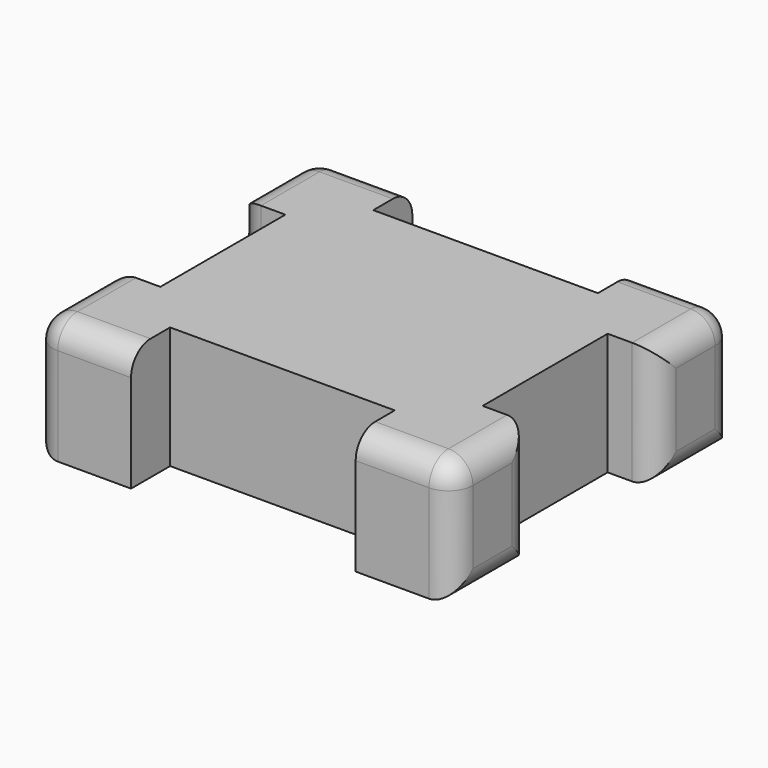
from build123d import *

# Parameters (mm, degrees)
F0_W         = 10
F0_H         = 10
F1_DEPTH     = 25
F2_T         = -2.5
F3_T1_DEPTH  = 27.5
F3_T3_DEPTH  = 27.5
F3_T5_DEPTH  = 27.5
F3_T7_DEPTH  = 27.5
F3_T9_DEPTH  = 32.5
F3_T11_DEPTH = 50
F3_T13_DEPTH = 45
F3_T15_DEPTH = 45
F3_S19_W     = 5
F3_S19_H     = 5
F3_T20_DEPTH = 5
F3_S25_W     = 5
F3_S25_H     = 5
F3_T26_DEPTH = 5
F3_S31_W     = 5
F3_S31_H     = 5
F3_T32_DEPTH = 5
F3_S37_W     = 5
F3_S37_H     = 5
F3_T38_DEPTH = 5


# Not quite as in the source:
# - a fillet or chamfer that OpenCascade refuses, or shapes differently, is made with other operations: its cross-section is extruded or revolved along the edge and cut away or added


with BuildPart() as f1:
    # F0 (on Top) → F1 (new body)
    with BuildSketch(Plane.XY):
        Polygon((-33, 16), (-33, 26), (-23, 26), (-23, 36), (-43, 36), (-43, 16), align=None)
        with Locations((-28, 21)):
            Rectangle(F0_W, F0_H)
        Polygon((23, 26), (-23, 26), (-23, 16), (-33, 16), (-33, -16), (-23, -16), (-23, -26), (23, -26), (23, -16), (33, -16), (33, 16), (23, 16), align=None)
        Polygon((23, 36), (23, 26), (33, 26), (33, 16), (43, 16), (43, 36), align=None)
        with Locations((28, 21)):
            Rectangle(F0_W, F0_H)
        with Locations((-28, -21)):
            Rectangle(F0_W, F0_H)
        Polygon((-33, -26), (-33, -16), (-43, -16), (-43, -36), (-23, -36), (-23, -26), align=None)
        Polygon((43, -16), (33, -16), (33, -26), (23, -26), (23, -36), (43, -36), align=None)
        with Locations((28, -21)):
            Rectangle(F0_W, F0_H)
    extrude(amount=F1_DEPTH)

    # F2
    f2_openings = [f1.faces().sort_by_distance(p)[0] for p in [
        (0, 0, 0),
    ]]
    offset(amount=F2_T, openings=f2_openings, kind=Kind.INTERSECTION)

    # F3: fillet of radius 5 on 20 edges, made by hand

    # F3_s2 → F3_t1 (cut)
    with BuildSketch(Plane.YZ.offset(-38)):
        with BuildLine():
            ThreePointArc((36, 20), (34.5355339059, 23.5355339059), (31, 25))
            Line((31, 25), (36, 25))
            Line((36, 25), (36, 20))
        make_face()
        with BuildLine():
            ThreePointArc((-36, 20), (-34.5355339059, 23.5355339059), (-31, 25))
            Line((-31, 25), (-36, 25))
            Line((-36, 25), (-36, 20))
        make_face()
    extrude(amount=F3_T1_DEPTH, mode=Mode.SUBTRACT)

    # F3_s4 → F3_t3 (cut)
    with BuildSketch(Plane.YZ.offset(10.5)):
        with BuildLine():
            ThreePointArc((-36, 20), (-34.5355339059, 23.5355339059), (-31, 25))
            Line((-31, 25), (-36, 25))
            Line((-36, 25), (-36, 20))
        make_face()
        with BuildLine():
            ThreePointArc((36, 20), (34.5355339059, 23.5355339059), (31, 25))
            Line((31, 25), (36, 25))
            Line((36, 25), (36, 20))
        make_face()
    extrude(amount=F3_T3_DEPTH, mode=Mode.SUBTRACT)

    # F3_s6 → F3_t5 (cut)
    with BuildSketch(Plane.XZ.offset(-31)):
        with BuildLine():
            ThreePointArc((43, 20), (41.5355339059, 23.5355339059), (38, 25))
            Line((38, 25), (43, 25))
            Line((43, 25), (43, 20))
        make_face()
        with BuildLine():
            ThreePointArc((-43, 20), (-41.5355339059, 23.5355339059), (-38, 25))
            Line((-38, 25), (-43, 25))
            Line((-43, 25), (-43, 20))
        make_face()
    extrude(amount=F3_T5_DEPTH, mode=Mode.SUBTRACT)

    # F3_s8 → F3_t7 (cut)
    with BuildSketch(Plane.XZ.offset(3.5)):
        with BuildLine():
            ThreePointArc((43, 20), (41.5355339059, 23.5355339059), (38, 25))
            Line((38, 25), (43, 25))
            Line((43, 25), (43, 20))
        make_face()
        with BuildLine():
            ThreePointArc((-43, 20), (-41.5355339059, 23.5355339059), (-38, 25))
            Line((-38, 25), (-43, 25))
            Line((-43, 25), (-43, 20))
        make_face()
    extrude(amount=F3_T7_DEPTH, mode=Mode.SUBTRACT)

    # F3_s10 → F3_t9 (cut)
    with BuildSketch(Plane.XY.offset(-12.5)):
        with BuildLine():
            ThreePointArc((-38, 36), (-41.5355339059, 34.5355339059), (-43, 31))
            Line((-43, 31), (-43, 36))
            Line((-43, 36), (-38, 36))
        make_face()
        with BuildLine():
            ThreePointArc((43, 31), (41.5355339059, 34.5355339059), (38, 36))
            Line((38, 36), (43, 36))
            Line((43, 36), (43, 31))
        make_face()
        with BuildLine():
            ThreePointArc((38, -36), (41.5355339059, -34.5355339059), (43, -31))
            Line((43, -31), (43, -36))
            Line((43, -36), (38, -36))
        make_face()
        with BuildLine():
            ThreePointArc((-43, -31), (-41.5355339059, -34.5355339059), (-38, -36))
            Line((-38, -36), (-43, -36))
            Line((-43, -36), (-43, -31))
        make_face()
    extrude(amount=F3_T9_DEPTH, mode=Mode.SUBTRACT)

    # F3_s12 → F3_t11 (cut)
    with BuildSketch(Plane.XY.offset(-12.5)):
        with BuildLine():
            ThreePointArc((-43, 21), (-41.5355339059, 17.4644660941), (-38, 16))
            Line((-38, 16), (-43, 16))
            Line((-43, 16), (-43, 21))
        make_face()
        with BuildLine():
            ThreePointArc((38, 16), (41.5355339059, 17.4644660941), (43, 21))
            Line((43, 21), (43, 16))
            Line((43, 16), (38, 16))
        make_face()
        with BuildLine():
            ThreePointArc((43, -21), (41.5355339059, -17.4644660941), (38, -16))
            Line((38, -16), (43, -16))
            Line((43, -16), (43, -21))
        make_face()
        with BuildLine():
            ThreePointArc((-38, -16), (-41.5355339059, -17.4644660941), (-43, -21))
            Line((-43, -21), (-43, -16))
            Line((-43, -16), (-38, -16))
        make_face()
    extrude(amount=F3_T11_DEPTH, mode=Mode.SUBTRACT)

    # F3_s14 → F3_t13 (cut)
    with BuildSketch(Plane.XZ.offset(-48.5)):
        with BuildLine():
            ThreePointArc((-43, 5), (-41.5355339059, 1.4644660941), (-38, 0))
            Line((-38, 0), (-43, 0))
            Line((-43, 0), (-43, 5))
        make_face()
        with BuildLine():
            ThreePointArc((43, 5), (41.5355339059, 1.4644660941), (38, 0))
            Line((38, 0), (43, 0))
            Line((43, 0), (43, 5))
        make_face()
    extrude(amount=F3_T13_DEPTH, mode=Mode.SUBTRACT)

    # F3_s16 → F3_t15 (cut)
    with BuildSketch(Plane.XZ.offset(3.5)):
        with BuildLine():
            ThreePointArc((43, 5), (41.5355339059, 1.4644660941), (38, 0))
            Line((38, 0), (43, 0))
            Line((43, 0), (43, 5))
        make_face()
        with BuildLine():
            ThreePointArc((-43, 5), (-41.5355339059, 1.4644660941), (-38, 0))
            Line((-38, 0), (-43, 0))
            Line((-43, 0), (-43, 5))
        make_face()
    extrude(amount=F3_T15_DEPTH, mode=Mode.SUBTRACT)


with BuildPart() as f3_tool18:
    # F3_s19 → F3_t20 (new body)
    with BuildSketch(Plane.XZ.offset(-31)):
        with Locations((-40.5, 22.5)):
            Rectangle(F3_S19_W, F3_S19_H)
    extrude(amount=-F3_T20_DEPTH)

    # F3_s21 → F3_t22 (revolve, cut)
    with BuildSketch(Plane(origin=(-38, 31, 20), x_dir=(0.7071067812, 0, -0.7071067812), z_dir=(0.7071067812, 0, 0.7071067812))):
        with BuildLine():
            ThreePointArc((0, -5), (5, 0), (0, 5))
            Line((0, 5), (0, -5))
        make_face()
    revolve(axis=Axis((-38, 31, 20), (0, 1, 0)), mode=Mode.SUBTRACT)


with BuildPart() as f1_1:
    add(f1.part)

    # F3_t17: cut F3_tool18
    add(f3_tool18.part, mode=Mode.SUBTRACT)


with BuildPart() as f3_tool24:
    # F3_s25 → F3_t26 (new body)
    with BuildSketch(Plane.XY.offset(20)):
        with Locations((-40.5, -33.5)):
            Rectangle(F3_S25_W, F3_S25_H)
    extrude(amount=F3_T26_DEPTH)

    # F3_s27 → F3_t28 (revolve, cut)
    with BuildSketch(Plane(origin=(-38, -31, 20), x_dir=(0.7071067812, 0.7071067812, 0), z_dir=(0.7071067812, -0.7071067812, 0))):
        with BuildLine():
            ThreePointArc((0, -5), (5, 0), (0, 5))
            Line((0, 5), (0, -5))
        make_face()
    revolve(axis=Axis((-38, -31, 20), (0, 0, 1)), mode=Mode.SUBTRACT)


with BuildPart() as f1_2:
    add(f1_1.part)

    # F3_t23: cut F3_tool24
    add(f3_tool24.part, mode=Mode.SUBTRACT)


with BuildPart() as f3_tool30:
    # F3_s31 → F3_t32 (new body)
    with BuildSketch(Plane.XZ.offset(31)):
        with Locations((40.5, 22.5)):
            Rectangle(F3_S31_W, F3_S31_H)
    extrude(amount=F3_T32_DEPTH)

    # F3_s33 → F3_t34 (revolve, cut)
    with BuildSketch(Plane(origin=(38, -31, 20), x_dir=(-0.7071067812, 0, -0.7071067812), z_dir=(-0.7071067812, 0, 0.7071067812))):
        with BuildLine():
            ThreePointArc((0, -5), (5, 0), (0, 5))
            Line((0, 5), (0, -5))
        make_face()
    revolve(axis=Axis((38, -31, 20), (0, -1, 0)), mode=Mode.SUBTRACT)


with BuildPart() as f1_3:
    add(f1_2.part)

    # F3_t29: cut F3_tool30
    add(f3_tool30.part, mode=Mode.SUBTRACT)


with BuildPart() as f3_tool36:
    # F3_s37 → F3_t38 (new body)
    with BuildSketch(Plane.XZ.offset(-31)):
        with Locations((40.5, 22.5)):
            Rectangle(F3_S37_W, F3_S37_H)
    extrude(amount=-F3_T38_DEPTH)

    # F3_s39 → F3_t40 (revolve, cut)
    with BuildSketch(Plane(origin=(38, 31, 20), x_dir=(-0.7071067812, 0, -0.7071067812), z_dir=(0.7071067812, 0, -0.7071067812))):
        with BuildLine():
            ThreePointArc((0, -5), (5, 0), (0, 5))
            Line((0, 5), (0, -5))
        make_face()
    revolve(axis=Axis((38, 31, 20), (0, 1, 0)), mode=Mode.SUBTRACT)


with BuildPart() as f1_4:
    add(f1_3.part)

    # F3_t35: cut F3_tool36
    add(f3_tool36.part, mode=Mode.SUBTRACT)


solid = f1_4.part
